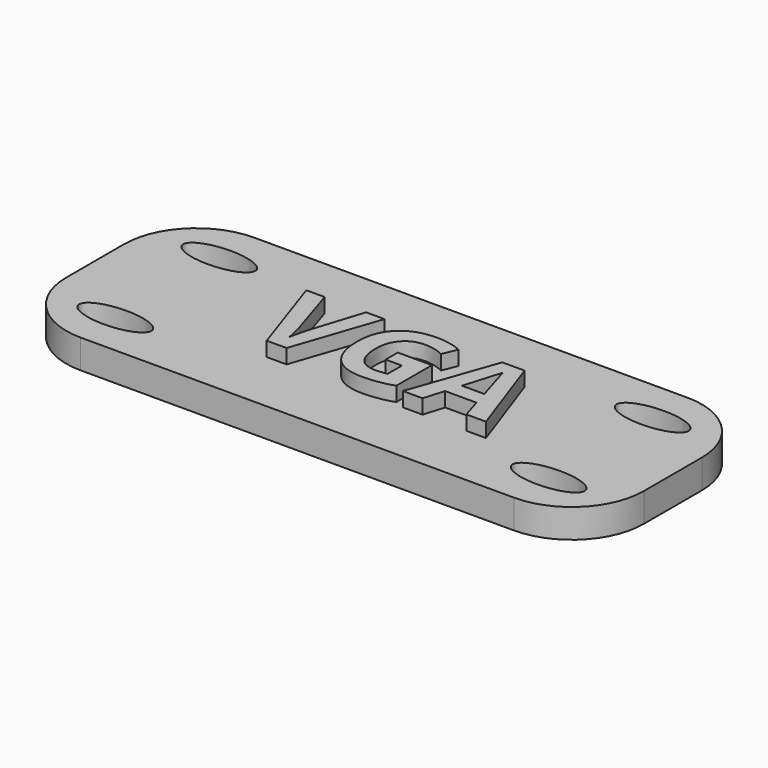
from build123d import *

# Parameters (mm, degrees)
F0_W         = 40
F0_H         = 15
F1_DEPTH     = 2
F2_TEXT_SIZE = 8.3333333333
F3_DEPTH     = 1
F4_R         = 5


# Not quite as in the source:
# - Text() gives the source's letters only with a copy of the font that has no kerning and outlines rounded to 1/6400 em; it was checked with that copy


with BuildPart() as f1:
    # F0 (on Top) → F1 (new body)
    with BuildSketch(Plane.XY):
        Rectangle(F0_W, F0_H)
        with BuildLine():
            add(Edge.make_bspline(
                [(-12.5, -4.5), (-12.5, -2.7679491924), (-16.25, -3.6339745962), (-20, -4.5), (-16.25, -5.3660254038), (-12.5, -6.2320508076), (-12.5, -4.5)],
                knots=[0, 0, 0, 2.0943951024, 2.0943951024, 4.1887902048, 4.1887902048, 6.2831853072, 6.2831853072, 6.2831853072], degree=2, weights=[1, 0.5, 1, 0.5, 1, 0.5, 1]))
        make_face(mode=Mode.SUBTRACT)
        with BuildLine():
            add(Edge.make_bspline(
                [(17.5, -4.5), (17.5, -2.7679491924), (13.75, -3.6339745962), (10, -4.5), (13.75, -5.3660254038), (17.5, -6.2320508076), (17.5, -4.5)],
                knots=[0, 0, 0, 2.0943951024, 2.0943951024, 4.1887902048, 4.1887902048, 6.2831853072, 6.2831853072, 6.2831853072], degree=2, weights=[1, 0.5, 1, 0.5, 1, 0.5, 1]))
        make_face(mode=Mode.SUBTRACT)
        with BuildLine():
            add(Edge.make_bspline(
                [(-12.5, 4.5), (-12.5, 6.2320508076), (-16.25, 5.3660254038), (-20, 4.5), (-16.25, 3.6339745962), (-12.5, 2.7679491924), (-12.5, 4.5)],
                knots=[0, 0, 0, 2.0943951024, 2.0943951024, 4.1887902048, 4.1887902048, 6.2831853072, 6.2831853072, 6.2831853072], degree=2, weights=[1, 0.5, 1, 0.5, 1, 0.5, 1]))
        make_face(mode=Mode.SUBTRACT)
        with BuildLine():
            add(Edge.make_bspline(
                [(17.5, 4.5), (17.5, 6.2320508076), (13.75, 5.3660254038), (10, 4.5), (13.75, 3.6339745962), (17.5, 2.7679491924), (17.5, 4.5)],
                knots=[0, 0, 0, 2.0943951024, 2.0943951024, 4.1887902048, 4.1887902048, 6.2831853072, 6.2831853072, 6.2831853072], degree=2, weights=[1, 0.5, 1, 0.5, 1, 0.5, 1]))
        make_face(mode=Mode.SUBTRACT)
    extrude(amount=F1_DEPTH)

    # F4
    f4_edges = [f1.edges().sort_by_distance(p)[0] for p in [
        (-20, 7.5, 1),
        (20, 7.5, 1),
        (-20, -7.5, 1),
        (20, -7.5, 1),
    ]]
    fillet(f4_edges, radius=F4_R)


with BuildPart() as f3:
    # F2 (on face) → F3 (new body)
    with BuildSketch(Plane.XY.offset(2)):
        with Locations((-7.7395833333, -3)):
            Text('VGA', F2_TEXT_SIZE, font='Open Sans', font_style=FontStyle.BOLD, text_align=(TextAlign.LEFT, TextAlign.BOTTOM))
    extrude(amount=F3_DEPTH)


solid = Compound([f1.part, f3.part])
